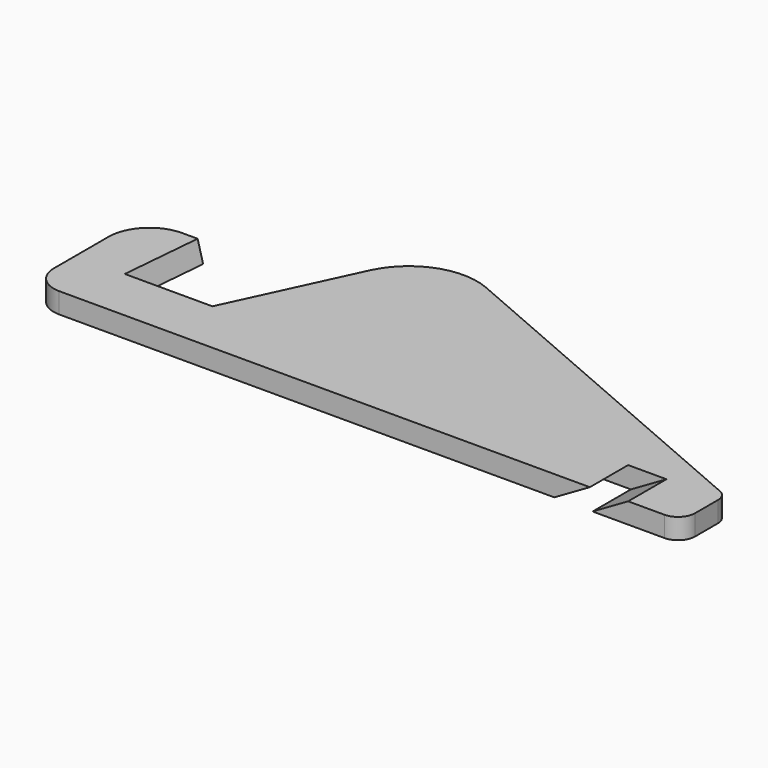
from build123d import *

# Parameters (mm, degrees)
F1_DEPTH = 3
F5_SIZE2 = 0.803838
F5_SIZE  = 2.99999
F4_W     = 7
F4_H     = 2.8
F6_DEPTH = 12.5


# Not quite as in the source:
# - a fillet or chamfer is up to 0.001 mm smaller than in the source, because OpenCascade refuses the exact size


with BuildPart() as f1:
    # F0 (on Top) → F1 (new body)
    with BuildSketch(Plane.XY):
        with BuildLine():
            Line((4, 0), (92.5, 0))
            ThreePointArc((92.5, 0), (94.267766953, 0.732233047), (95, 2.5))
            Line((95, 2.5), (95, 6.6861086512))
            ThreePointArc((95, 6.6861086512), (94.6715622153, 7.784234218), (93.7941202395, 8.5216938563))
            Line((93.7941202395, 8.5216938563), (41.5145959947, 31.1391284496))
            ThreePointArc((41.5145959947, 31.1391284496), (33.9924781689, 31.3092893749), (28.4809169267, 26.1873850415))
            Line((28.4809169267, 26.1873850415), (20, 8))
            Line((20, 8), (8, 8))
            Line((8, 8), (9.0498639623, 20))
            Line((9.0498639623, 20), (6, 20))
            ThreePointArc((6, 20), (1.7573593129, 18.2426406871), (0, 14))
            Line((0, 14), (0, 4))
            ThreePointArc((0, 4), (1.1715728753, 1.1715728753), (4, 0))
        make_face()
    extrude(amount=F1_DEPTH)

    # F5 (size 3 and 0.8038475773 in the source; OpenCascade refuses exactly that, so slightly less here)
    f5_edges = [f1.edges().sort_by_distance(p)[0] for p in [
        (8.524932, 14, 3),
    ]]
    f5_side = f1.faces().sort_by_distance((8.524932, 14, 1.5))[0]
    chamfer(f5_edges, length=F5_SIZE, length2=F5_SIZE2, reference=f5_side)

    # F4 (on line) → F6 (cut, symmetric)
    with BuildSketch(Plane(origin=(61.5, 0, 35.5070415552), x_dir=(0, 1, 0), z_dir=(0.8660254038, 0, 0.5))):
        with Locations((3.5, -39.6)):
            Rectangle(F4_W, F4_H)
    extrude(amount=F6_DEPTH, both=True, mode=Mode.SUBTRACT)


solid = f1.part
